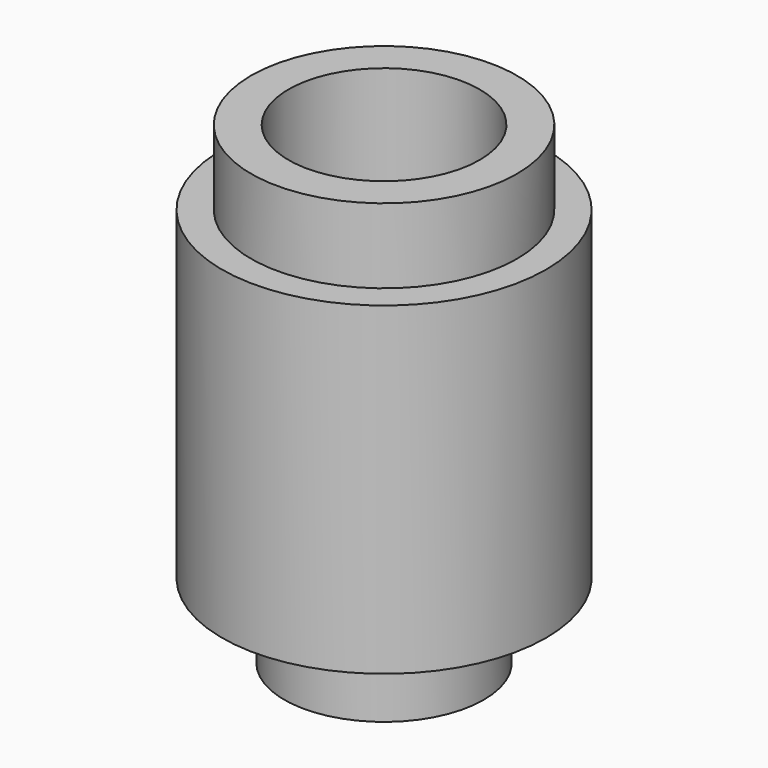
from build123d import *

# Parameters (mm, degrees)
F0_R     = 2.4
F1_DEPTH = 1.8
F2_R     = 3.9
F2_R_2   = 2.4
F3_DEPTH = 9.6
F4_R     = 3.9
F4_R_2   = 3.2
F5_DEPTH = 1.8
F6_R     = 2.3
F7_DEPTH = 8.8
F8_R     = 1.6
F9_DEPTH = 1.8


# Not quite as in the source:
# - a feature names something its author has since deleted; it is built from what else it names


with BuildPart() as f1:
    # F0 (on Top) → F1 (new body)
    with BuildSketch(Plane.XY):
        Circle(F0_R)
    extrude(amount=F1_DEPTH)

    # F2 (on face) → F3 (join)
    with BuildSketch(Plane.XY.offset(1.8)):
        Circle(F2_R)
        Circle(F2_R_2, mode=Mode.SUBTRACT)
        Circle(F2_R_2)
    extrude(amount=F3_DEPTH)

    # F4 (on face) → F5 (cut)
    with BuildSketch(Plane.XY.offset(11.4)):
        Circle(F4_R)
        Circle(F4_R_2, mode=Mode.SUBTRACT)
    extrude(amount=-F5_DEPTH, mode=Mode.SUBTRACT)

    # F6 (on face) → F7 (cut)
    with BuildSketch(Plane.XY.offset(11.4)):
        Circle(F6_R)
    extrude(amount=-F7_DEPTH, mode=Mode.SUBTRACT)

    # F8 (on face) → F9 (cut)
    with BuildSketch(Plane.XY.offset(2.6)):
        Circle(F8_R)
    extrude(amount=-F9_DEPTH, mode=Mode.SUBTRACT)


solid = f1.part
